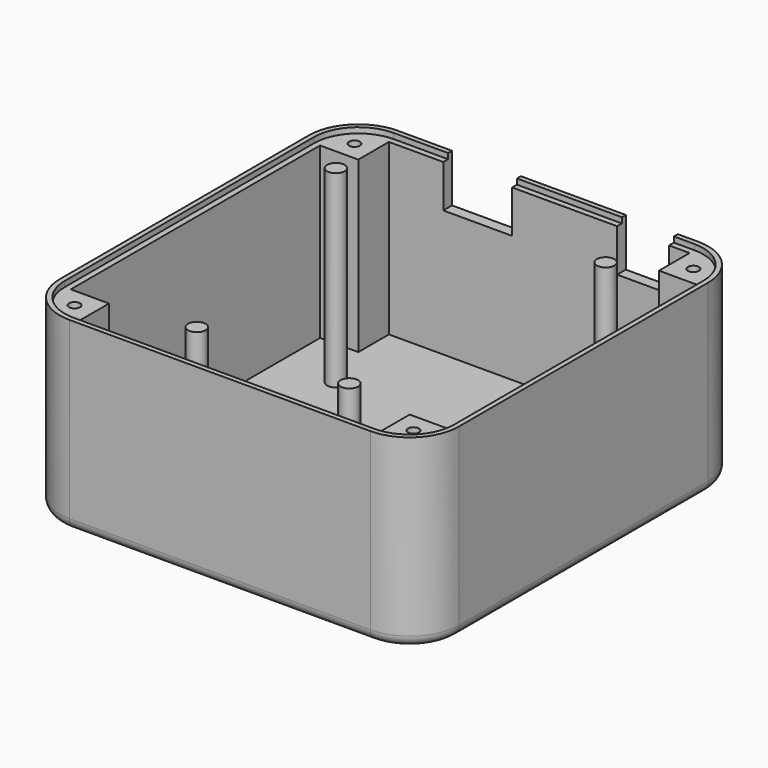
from build123d import *

# Parameters (mm, degrees)
F1_DEPTH      = 2
F2_R          = 1.6
F3_DEPTH      = 34.5
F5_DEPTH      = 32
F7_DEPTH      = 1
F8_W          = 12.6
F8_H          = 2
F8_W_2        = 9.5
F9_DEPTH      = 8.8
F11_DEPTH     = 31
F12_R         = 1
F13_DEPTH     = 7
F14_R         = 2
F15_TEXT_SIZE = 8.8728524538
F16_DEPTH     = 0.5


# Not quite as in the source:
# - Text() gives the source's letters only with a copy of the font that has no kerning and outlines rounded to 1/6400 em; it was checked with that copy


with BuildPart() as f1:
    # F0 (on Top) → F1 (new body)
    with BuildSketch(Plane.XY):
        with BuildLine():
            Line((27.5, 38.5), (-27.5, 38.5))
            ThreePointArc((-27.5, 38.5), (-33.8639610307, 35.8639610307), (-36.5, 29.5))
            Line((-36.5, 29.5), (-36.5, -27.5))
            ThreePointArc((-36.5, -27.5), (-33.8639610307, -33.8639610307), (-27.5, -36.5))
            Line((-27.5, -36.5), (27.5, -36.5))
            ThreePointArc((27.5, -36.5), (33.8639610307, -33.8639610307), (36.5, -27.5))
            Line((36.5, -27.5), (36.5, 29.5))
            ThreePointArc((36.5, 29.5), (33.8639610307, 35.8639610307), (27.5, 38.5))
        make_face()
    extrude(amount=F1_DEPTH)

    # F2 (on face) → F3 (join)
    with BuildSketch(Plane.XY.offset(2)):
        with Locations((-24.16, 20.2)):
            Circle(F2_R)
        with Locations((24.14, 21.5)):
            Circle(F2_R)
        with Locations((18.94, -30.6)):
            Circle(F2_R)
        with Locations((-8.96, -30.6)):
            Circle(F2_R)
    extrude(amount=F3_DEPTH)

    # F4 (on face) → F5 (join)
    with BuildSketch(Plane.XY.offset(2)):
        with BuildLine():
            Line((27.5, 38.5), (-27.5, 38.5))
            ThreePointArc((-27.5, 38.5), (-33.8639610307, 35.8639610307), (-36.5, 29.5))
            Line((-36.5, 29.5), (-36.5, -27.5))
            ThreePointArc((-36.5, -27.5), (-33.8639610307, -33.8639610307), (-27.5, -36.5))
            Line((-27.5, -36.5), (27.5, -36.5))
            ThreePointArc((27.5, -36.5), (33.8639610307, -33.8639610307), (36.5, -27.5))
            Line((36.5, -27.5), (36.5, 29.5))
            ThreePointArc((36.5, 29.5), (33.8639610307, 35.8639610307), (27.5, 38.5))
        make_face()
        with BuildLine():
            ThreePointArc((-34.5, 29.5), (-32.4497474683, 34.4497474683), (-27.5, 36.5))
            Line((-27.5, 36.5), (27.5, 36.5))
            ThreePointArc((27.5, 36.5), (32.4497474683, 34.4497474683), (34.5, 29.5))
            Line((34.5, 29.5), (34.5, -27.5))
            ThreePointArc((34.5, -27.5), (32.4497474683, -32.4497474683), (27.5, -34.5))
            Line((27.5, -34.5), (-27.5, -34.5))
            ThreePointArc((-27.5, -34.5), (-32.4497474683, -32.4497474683), (-34.5, -27.5))
            Line((-34.5, -27.5), (-34.5, 29.5))
        make_face(mode=Mode.SUBTRACT)
    extrude(amount=F5_DEPTH)

    # F6 (on face) → F7 (cut)
    with BuildSketch(Plane.XY.offset(34)):
        with BuildLine():
            Line((27.5, 37.6), (-27.5, 37.6))
            ThreePointArc((-27.5, 37.6), (-33.2275649276, 35.2275649276), (-35.6, 29.5))
            Line((-35.6, 29.5), (-35.6, -27.5))
            ThreePointArc((-35.6, -27.5), (-33.2275649276, -33.2275649276), (-27.5, -35.6))
            Line((-27.5, -35.6), (27.5, -35.6))
            ThreePointArc((27.5, -35.6), (33.2275649276, -33.2275649276), (35.6, -27.5))
            Line((35.6, -27.5), (35.6, 29.5))
            ThreePointArc((35.6, 29.5), (33.2275649276, 35.2275649276), (27.5, 37.6))
        make_face()
        with BuildLine():
            ThreePointArc((-34.5, 29.5), (-32.4497474683, 34.4497474683), (-27.5, 36.5))
            Line((-27.5, 36.5), (27.5, 36.5))
            ThreePointArc((27.5, 36.5), (32.4497474683, 34.4497474683), (34.5, 29.5))
            Line((34.5, 29.5), (34.5, -27.5))
            ThreePointArc((34.5, -27.5), (32.4497474683, -32.4497474683), (27.5, -34.5))
            Line((27.5, -34.5), (-27.5, -34.5))
            ThreePointArc((-27.5, -34.5), (-32.4497474683, -32.4497474683), (-34.5, -27.5))
            Line((-34.5, -27.5), (-34.5, 29.5))
        make_face(mode=Mode.SUBTRACT)
    extrude(amount=-F7_DEPTH, mode=Mode.SUBTRACT)

    # F8 (on face) → F9 (cut)
    with BuildSketch(Plane.XY.offset(34)):
        with Locations((-11.26, 37.5)):
            Rectangle(F8_W, F8_H)
        with Locations((18.99, 37.5)):
            Rectangle(F8_W_2, F8_H)
    extrude(amount=-F9_DEPTH, mode=Mode.SUBTRACT)

    # F10 (on face) → F11 (join)
    with BuildSketch(Plane.XY.offset(2)):
        with BuildLine():
            Line((-27.5, 29.5), (-27.5, 36.5))
            ThreePointArc((-27.5, 36.5), (-32.4497474683, 34.4497474683), (-34.5, 29.5))
            Line((-34.5, 29.5), (-27.5, 29.5))
        make_face()
        with BuildLine():
            Line((27.5, 29.5), (34.5, 29.5))
            ThreePointArc((34.5, 29.5), (32.4497474683, 34.4497474683), (27.5, 36.5))
            Line((27.5, 36.5), (27.5, 29.5))
        make_face()
        with BuildLine():
            Line((27.5, -27.5), (27.5, -34.5))
            ThreePointArc((27.5, -34.5), (32.4497474683, -32.4497474683), (34.5, -27.5))
            Line((34.5, -27.5), (27.5, -27.5))
        make_face()
        with BuildLine():
            Line((-27.5, -27.5), (-34.5, -27.5))
            ThreePointArc((-34.5, -27.5), (-32.4497474683, -32.4497474683), (-27.5, -34.5))
            Line((-27.5, -34.5), (-27.5, -27.5))
        make_face()
    extrude(amount=F11_DEPTH)

    # F12 (on face) → F13 (cut)
    with BuildSketch(Plane.XY.offset(33)):
        with Locations((-31, 33)):
            Circle(F12_R)
        with Locations((31, 33)):
            Circle(F12_R)
        with Locations((31, -31)):
            Circle(F12_R)
        with Locations((-31, -31)):
            Circle(F12_R)
    extrude(amount=-F13_DEPTH, mode=Mode.SUBTRACT)

    # F14
    f14_edges = [f1.edges().sort_by_distance(p)[0] for p in [
        (0, 38.5, 0),
    ]]
    fillet(f14_edges, radius=F14_R)

    # F15 (on face) → F16 (join)
    with BuildSketch(Plane(origin=(0, 0, 0), x_dir=(1, 0, 0), z_dir=(0, 0, -1))):
        with Locations((-25.5853352815, -21.0167699605)):
            Text('wind station', F15_TEXT_SIZE, font='Open Sans', text_align=(TextAlign.LEFT, TextAlign.BOTTOM))
    extrude(amount=F16_DEPTH)


solid = f1.part
